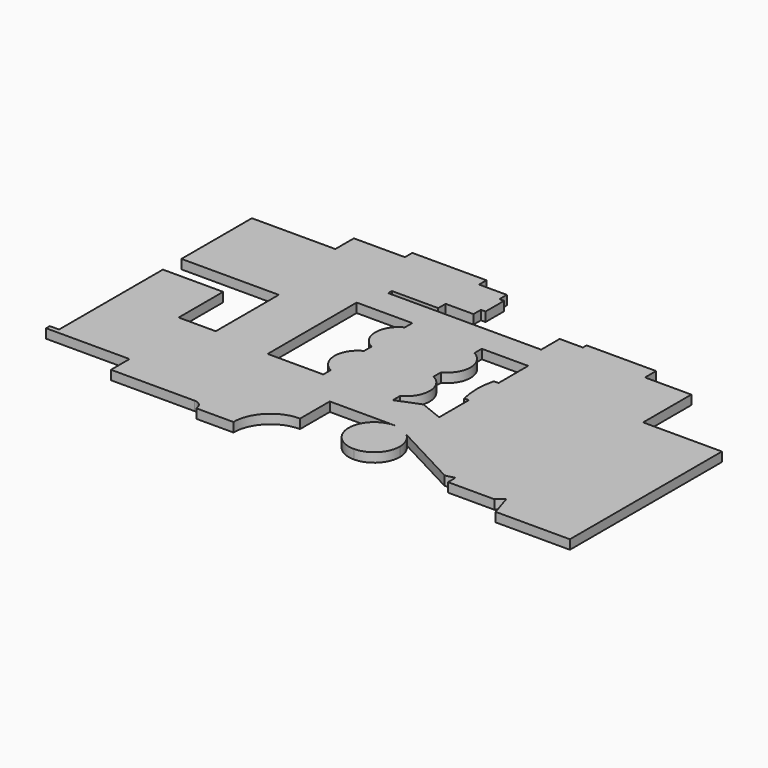
from build123d import *

# Parameters (mm, degrees)
F1_DEPTH = 3.175


# Not quite as in the source:
# - ends of sketch curves that miss each other by under 0.0002 mm in the source are joined


with BuildPart() as f1:
    # F0 (on Top) → F1 (new body)
    with BuildSketch(Plane.XY):
        with BuildLine():
            Line((-34.925, 35.7325066477), (-55.5625, 35.7325066477))
            Line((-55.5625, 35.7325066477), (-55.5625, -8.7174933523))
            Line((-55.5625, -8.7174933523), (-58.7375, -8.7174933523))
            Line((-58.7375, -8.7174933523), (-58.7375, -10.3049933523))
            Line((-58.7375, -10.3049933523), (-30.1625, -10.3049933523))
            Line((-30.1625, -10.3049933523), (-30.1625, -18.2424933523))
            Line((-30.1625, -18.2424933523), (-1.5875, -18.2424933523))
            ThreePointArc((-1.5875, -18.2424933523), (0.6575640303, -19.172429322), (1.5875, -21.4174933523))
            Line((1.5875, -21.4174933523), (14.2875, -21.4174933523))
            ThreePointArc((14.2875, -21.4174933523), (18.0072438789, -12.4372372312), (26.9875, -8.7174933523))
            Line((26.9875, -8.7174933523), (26.9875, 3.9825066477))
            Line((26.9875, 3.9825066477), (49.2125, 3.9825066477))
            ThreePointArc((49.2125, 3.9825066477), (52.3581189283, 3.3961819464), (55.0812659129, 1.7159541056))
            Line((55.0812659129, 1.7159541056), (77.7875, -10.3049933523))
            Line((77.7875, -10.3049933523), (80.8780316716, -9.5775052173))
            Line((80.8780316716, -9.5775052173), (80.8780316716, -12.7525052173))
            Line((80.8780316716, -12.7525052173), (96.7530316716, -12.7525052173))
            Line((96.7530316716, -12.7525052173), (99.1648957133, -10.6876718476))
            Line((99.1648957133, -10.6876718476), (101.6, -18.2424933523))
            Line((101.6, -18.2424933523), (104.775, -18.2424933523))
            Line((104.775, -18.2424933523), (119.0625, -18.2424933523))
            Line((119.0625, -18.2424933523), (127, -18.2424933523))
            Line((127, -18.2424933523), (127, 46.8450066477))
            Line((127, 46.8450066477), (100.0125, 46.8450066477))
            Line((100.0125, 46.8450066477), (100.0125, 67.4825066477))
            Line((100.0125, 67.4825066477), (84.1375, 67.4825066477))
            Line((84.1375, 67.4825066477), (84.1375, 72.2450066477))
            Line((84.1375, 72.2450066477), (66.675, 72.2450066477))
            Line((66.675, 72.2450066477), (60.325, 72.2450066477))
            Line((60.325, 72.2450066477), (60.325, 70.6575066477))
            Line((60.325, 70.6575066477), (52.3875, 70.6575066477))
            Line((52.3875, 70.6575066477), (52.3875, 62.7200066477))
            Line((52.3875, 62.7200066477), (0, 62.7200066477))
            Line((0, 62.7200066477), (0, 64.3075066477))
            Line((0, 64.3075066477), (15.875, 64.3075066477))
            Line((15.875, 64.3075066477), (15.875, 67.4825066477))
            Line((15.875, 67.4825066477), (25.4, 67.4825066477))
            Line((25.4, 67.4825066477), (25.4, 70.6575066477))
            Line((25.4, 70.6575066477), (26.9875, 70.6575066477))
            Line((26.9875, 70.6575066477), (26.9875, 78.5950066477))
            Line((26.9875, 78.5950066477), (25.4, 78.5950066477))
            Line((25.4, 78.5950066477), (25.4, 81.7700066477))
            Line((25.4, 81.7700066477), (15.875, 81.7700066477))
            Line((15.875, 81.7700066477), (15.875, 84.9450066477))
            Line((15.875, 84.9450066477), (-9.525, 84.9450066477))
            Line((-9.525, 84.9450066477), (-9.525, 81.7700066477))
            Line((-9.525, 81.7700066477), (-26.9875, 81.7700066477))
            Line((-26.9875, 81.7700066477), (-26.9875, 73.8325066477))
            Line((-26.9875, 73.8325066477), (-55.5625, 73.8325066477))
            Line((-55.5625, 73.8325066477), (-55.5625, 43.6700066477))
            Line((-55.5625, 43.6700066477), (-22.225, 43.6700066477))
            Line((-22.225, 43.6700066477), (-22.225, 16.6825066477))
            Line((-22.225, 16.6825066477), (-34.925, 16.6825066477))
            Line((-34.925, 16.6825066477), (-34.925, 35.7325066477))
        make_face()
        Polygon((-3.175, 53.1950066477), (15.875, 53.1950066477), (15.875, 50.0200066477), (15.875, 35.7325066477), (15.875, 32.5575066477), (15.875, 18.2700066477), (15.875, 15.0950066477), (-3.175, 15.0950066477), align=None, mode=Mode.SUBTRACT)
        Polygon((39.6875, 50.0200066477), (39.6875, 53.1950066477), (55.5625, 53.1950066477), (55.5625, 40.4950066477), (55.5625, 27.7950066477), (55.5625, 15.0950066477), (47.625, 18.2700066477), (39.6875, 15.0950066477), (39.6875, 18.2700066477), (39.6875, 32.5575066477), (39.6875, 35.7325066477), align=None, mode=Mode.SUBTRACT)
        with BuildLine():
            Line((15.875, 35.7325066477), (15.875, 50.0200066477))
            ThreePointArc((15.875, 50.0200066477), (11.4771704008, 42.8762566477), (15.875, 35.7325066477))
        make_face()
        with BuildLine():
            Line((15.875, 18.2700066477), (15.875, 32.5575066477))
            ThreePointArc((15.875, 32.5575066477), (11.4771704008, 25.4137566477), (15.875, 18.2700066477))
        make_face()
        with BuildLine():
            ThreePointArc((39.6875, 35.7325066477), (44.0853295992, 42.8762566477), (39.6875, 50.0200066477))
            Line((39.6875, 50.0200066477), (39.6875, 35.7325066477))
        make_face()
        with BuildLine():
            ThreePointArc((39.6875, 18.2700066477), (44.0853295992, 25.4137566477), (39.6875, 32.5575066477))
            Line((39.6875, 32.5575066477), (39.6875, 18.2700066477))
        make_face()
        with BuildLine():
            Line((55.5625, 27.7950066477), (55.5625, 40.4950066477))
            Line((55.5625, 40.4950066477), (53.975, 40.4950066477))
            ThreePointArc((53.975, 40.4950066477), (53.1818915421, 34.1450066477), (53.975, 27.7950066477))
            Line((53.975, 27.7950066477), (55.5625, 27.7950066477))
        make_face()
        with BuildLine():
            ThreePointArc((55.0812659129, 1.7159541056), (52.3581189283, 3.3961819464), (49.2125, 3.9825066477))
            Line((49.2125, 3.9825066477), (49.2125, -13.4799933523))
            ThreePointArc((49.2125, -13.4799933523), (55.3864260832, -10.9226694355), (57.94375, -4.7487433523))
            ThreePointArc((57.94375, -4.7487433523), (57.1961203861, -1.2136999165), (55.0812659129, 1.7159541056))
        make_face()
        with BuildLine():
            Line((49.2125, -13.4799933523), (49.2125, 3.9825066477))
            ThreePointArc((49.2125, 3.9825066477), (40.48125, -4.7487433523), (49.2125, -13.4799933523))
        make_face()
    extrude(amount=F1_DEPTH)


solid = f1.part
